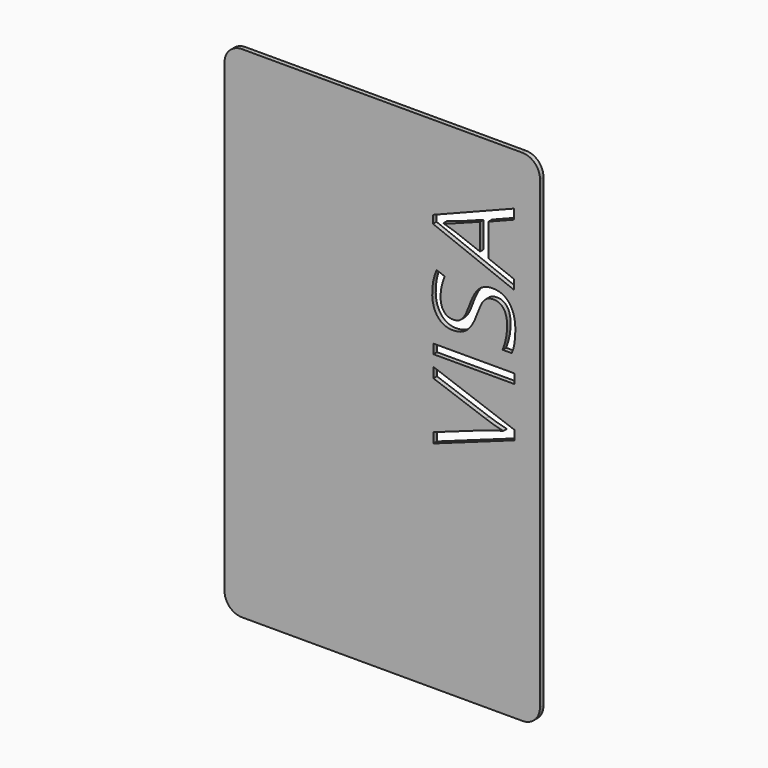
from build123d import *

# Parameters (mm, degrees)
F1_DEPTH     = 0.76
F2_TEXT_SIZE = 19.3921095763
F3_DEPTH     = 0.761


# Not quite as in the source:
# - Text() gives the source's letters only with a copy of the font that has no kerning and outlines rounded to 1/6400 em; it was checked with that copy


with BuildPart() as f1:
    # F0 (on Front) → F1 (new body)
    with BuildSketch(Plane.XZ):
        with BuildLine():
            Line((-50.98, 0), (-3, 0))
            ThreePointArc((-3, 0), (-0.8786796564, 0.8786796564), (0, 3))
            Line((0, 3), (0, 82.6))
            ThreePointArc((0, 82.6), (-0.8786796564, 84.7213203436), (-3, 85.6))
            Line((-3, 85.6), (-50.98, 85.6))
            ThreePointArc((-50.98, 85.6), (-53.1013203436, 84.7213203436), (-53.98, 82.6))
            Line((-53.98, 82.6), (-53.98, 3))
            ThreePointArc((-53.98, 3), (-53.1013203436, 0.8786796564), (-50.98, 0))
        make_face()
    extrude(amount=F1_DEPTH)

    # F2 (on face) → F3 (cut, through all)
    with BuildSketch(Plane.XZ.offset(0.76)):
        with Locations(Location((-4.3770074844, 36.8590094149), (0, 0, 90.057207811))):
            Text('VISA', F2_TEXT_SIZE, font='Open Sans', text_align=(TextAlign.LEFT, TextAlign.BOTTOM))
    extrude(amount=-F3_DEPTH, mode=Mode.SUBTRACT)


solid = f1.part
